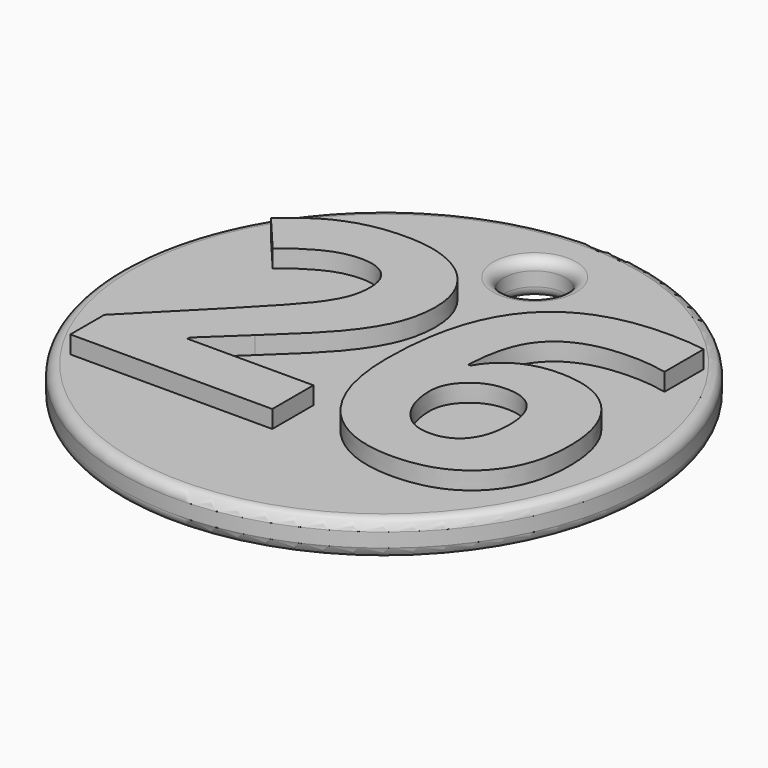
from build123d import *

# Parameters (mm, degrees)
F0_R         = 15
F1_DEPTH     = 2
F2_R         = 1.75
F3_DEPTH     = 2.001
F4_R         = 0.6
F5_TEXT_SIZE = 22.9912916585
F6_DEPTH     = 1


# Not quite as in the source:
# - Text() gives the source's letters only with a copy of the font that has no kerning and outlines rounded to 1/6400 em; it was checked with that copy


with BuildPart() as f1:
    # F0 (on Top) → F1 (new body)
    with BuildSketch(Plane.XY):
        Circle(F0_R)
    extrude(amount=F1_DEPTH)

    # F2 (on face) → F3 (cut, through all)
    with BuildSketch(Plane.XY.offset(2)):
        with Locations((0, 10.7)):
            Circle(F2_R)
    extrude(amount=-F3_DEPTH, mode=Mode.SUBTRACT)

    # F4
    f4_edges = [f1.edges().sort_by_distance(p)[0] for p in [
        (-15, 0, 2),
        (-1.75, 10.7, 2),
        (-1.75, 10.7, 0),
        (-15, 0, 0),
    ]]
    fillet(f4_edges, radius=F4_R)

    # F5 (on face) → F6 (join)
    with BuildSketch(Plane.XY.offset(2)):
        with Locations((-12.3665539008, -7.9758107806)):
            Text('2', F5_TEXT_SIZE, font='Open Sans', font_style=FontStyle.BOLD, text_align=(TextAlign.LEFT, TextAlign.BOTTOM))
        with Locations((0.1494788553, -7.9758107806)):
            Text('6', F5_TEXT_SIZE, font='Open Sans', font_style=FontStyle.BOLD, text_align=(TextAlign.LEFT, TextAlign.BOTTOM))
    extrude(amount=F6_DEPTH)


solid = f1.part
